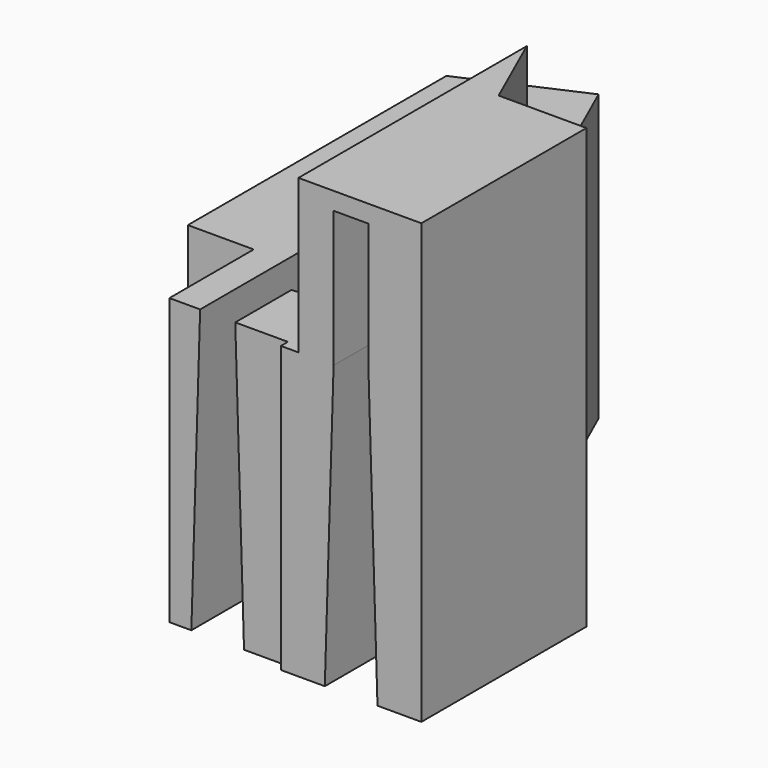
from build123d import *

# Parameters (mm, degrees)
F1_DEPTH     = 16.25
F2_DEPTH     = 25
F3_START     = 24
F3_DEPTH     = 1
F4_START     = 17
F4_DEPTH     = 8
F5_T1_DEPTH  = 88.2485217467
F5_T3_DEPTH  = 96.2485217467
F5_T5_DEPTH  = 88.9985217467
F5_T10_DEPTH = 96.5839074706
F5_T15_DEPTH = 88.4985217467
F5_T20_DEPTH = 86.4985217467
F5_T23_ANGLE = 359.64
F5_T25_ANGLE = 359.64


# Not quite as in the source:
# - a fillet or chamfer that OpenCascade refuses, or shapes differently, is made with other operations: its cross-section is extruded or revolved along the edge and cut away or added


with BuildPart() as f1:
    # F0 (on Top) → F1 (new body)
    with BuildSketch(Plane.XY):
        with BuildLine():
            Line((-8.75, -5.75), (-7, -5.75))
            Line((-7, -5.75), (-7, 6.3353857239))
            Line((-7, 6.3353857239), (-9.0223743914, 8.3577601154))
            Line((-9.0223743914, 8.3577601154), (-9.0223743914, 14.1793463062))
            Line((-9.0223743914, 14.1793463062), (-5.6981157623, 15.6555524338))
            Line((-5.6981157623, 15.6555524338), (-1.1670593175, 5.4520969645))
            Line((-1.1670593175, 5.4520969645), (-5, 3.75))
            Line((-5, 3.75), (-5, 1.75))
            ThreePointArc((-5, 1.75), (-3.7625631329, 1.2374368671), (-3.25, 0))
            ThreePointArc((-3.25, 0), (-3.7625631329, -1.2374368671), (-5, -1.75))
            Line((-5, -1.75), (-5, -5.75))
            Line((-5, -5.75), (-2, -5.75))
            Line((-2, -5.75), (-2, -6.25))
            Line((-2, -6.25), (-1, -6.25))
            Line((-1, -6.25), (-1, 10.0037865203))
            Line((-1, 10.0037865203), (-6.1024322628, 21.4939193431))
            Line((-6.1024322628, 21.4939193431), (-12.5, 18.652946438))
            Line((-12.5, 18.652946438), (-12.5, 0.25))
            Line((-12.5, 0.25), (-8.75, 0.25))
            Line((-8.75, 0.25), (-8.75, -5.75))
        make_face()
    extrude(amount=F1_DEPTH)

    # F0 (on Top) → F2 (join)
    with BuildSketch(Plane.XY):
        Polygon((1, 5.5), (-1, 10.0037865203), (-1, -6.25), (1, -6.25), align=None)
    extrude(amount=F2_DEPTH)



with BuildPart() as f2:
    # F0 (on Top) → F2, piece 2 (new body)
    with BuildSketch(Plane.XY):
        with BuildLine():
            Line((6, 5.5), (3, 5.5))
            Line((3, 5.5), (3, 1.75))
            ThreePointArc((3, 1.75), (4.75, 0), (3, -1.75))
            Line((3, -1.75), (3, -6.25))
            Line((3, -6.25), (6, -6.25))
            Line((6, -6.25), (6, 5.5))
        make_face()
    extrude(amount=F2_DEPTH)


with BuildPart() as f1_1:
    add(f1.part)

    add(f2.part)  # F3 merges F2
    # F0 (on Top) → F3 (join)
    with BuildSketch(Plane.XY.offset(F3_START)):
        Polygon((3, 5.5), (1, 5.5), (1, -6.25), (3, -6.25), (3, -1.75), (3, 1.75), align=None)
    extrude(amount=F3_DEPTH)

    # F0 (on Top) → F4 (join)
    with BuildSketch(Plane.XY.offset(F4_START)):
        with BuildLine():
            ThreePointArc((3, -1.75), (4.75, 0), (3, 1.75))
            Line((3, 1.75), (3, -1.75))
        make_face()
    extrude(amount=F4_DEPTH)

    # F5: chamfer of 16.25 x 0.5 on 8 edges, made by hand

    # F5_s2 → F5_t1 (cut)
    with BuildSketch(Plane.XZ.offset(-47.7492608733)):
        Polygon((3.5, 0), (3, 16.25), (3, 0), align=None)
    extrude(amount=F5_T1_DEPTH, mode=Mode.SUBTRACT)

    # F5_s4 → F5_t3 (cut)
    with BuildSketch(Plane.XZ.offset(-47.7492608733)):
        Polygon((0.5, 0), (1, 16.25), (1, 0), align=None)
    extrude(amount=F5_T3_DEPTH, mode=Mode.SUBTRACT)

    # F5_s6 → F5_t5 (cut)
    with BuildSketch(Plane.XZ.offset(-40.4992608733)):
        Polygon((3.5, 0), (3, 16.25), (3, 0), align=None)
    extrude(amount=F5_T5_DEPTH, mode=Mode.SUBTRACT)


with BuildPart() as f5_tool8:
    # F5_s9 → F5_t10 (new body)
    with BuildSketch(Plane.XZ.offset(47.9992608733)):
        Polygon((-7, 16.25), (-7.5, 0), (-7, 0), align=None)
    extrude(amount=-F5_T10_DEPTH)

    split(bisect_by=Plane(origin=(-0.332307138, -0.332307138, 0), x_dir=(0, 0, 1), z_dir=(-0.7071067812, -0.7071067812, 0)), keep=Keep.TOP)


with BuildPart() as f1_2:
    add(f1_1.part)

    # F5_t7: cut F5_tool8
    add(f5_tool8.part, mode=Mode.SUBTRACT)


with BuildPart() as f5_tool13:
    # F5_s14 → F5_t15 (new body)
    with BuildSketch(Plane.XZ.offset(-40.4992608733)):
        Polygon((-5, 16.25), (-4.5, 0), (-5, 0), align=None)
    extrude(amount=F5_T15_DEPTH)

    split(bisect_by=Plane(origin=(1.0474931823, 0.4651611161, 0), x_dir=(0, 0, 1), z_dir=(-0.9139382482, -0.4058532722, 0)), keep=Keep.TOP)


with BuildPart() as f1_3:
    add(f1_2.part)

    # F5_t12: cut F5_tool13
    add(f5_tool13.part, mode=Mode.SUBTRACT)


with BuildPart() as f5_tool18:
    # F5_s19 → F5_t20 (new body)
    with BuildSketch(Plane.XZ.offset(-45.9992608733)):
        Polygon((-5, 16.25), (-4.5, 0), (-5, 0), align=None)
    extrude(amount=F5_T20_DEPTH)

    split(bisect_by=Plane(origin=(1.0474931823, 0.4651611161, 0), x_dir=(0, 0, 1), z_dir=(-0.9139382482, -0.4058532722, 0)), keep=Keep.TOP)


with BuildPart() as f1_4:
    add(f1_3.part)

    # F5_t17: cut F5_tool18
    add(f5_tool18.part, mode=Mode.SUBTRACT)

    # F5_s22 → F5_t23 (revolve, cut)
    with BuildSketch(Plane(origin=(-4.93479e-05, -0.0157078599, 0), x_dir=(0, 0, 1), z_dir=(-0.0031415875, -0.9999950652, 0))):
        Polygon((16.25, 6.749975326), (0, 7.249975326), (0, 6.749975326), align=None)
    revolve(axis=Axis((-5, 0, 0), (0, 0, -1)), revolution_arc=F5_T23_ANGLE, mode=Mode.SUBTRACT)

    # F5_s24 → F5_t25 (revolve, cut)
    with BuildSketch(Plane(origin=(2.96087e-05, 0.0094247159, 0), x_dir=(0, 0, 1), z_dir=(-0.0031415875, -0.9999950652, 0))):
        Polygon((0, -0.7499851956), (16.25, -1.2499851956), (0, -1.2499851956), align=None)
    revolve(axis=Axis((3, 0, 0), (0, 0, -1)), revolution_arc=F5_T25_ANGLE, mode=Mode.SUBTRACT)


solid = f1_4.part
